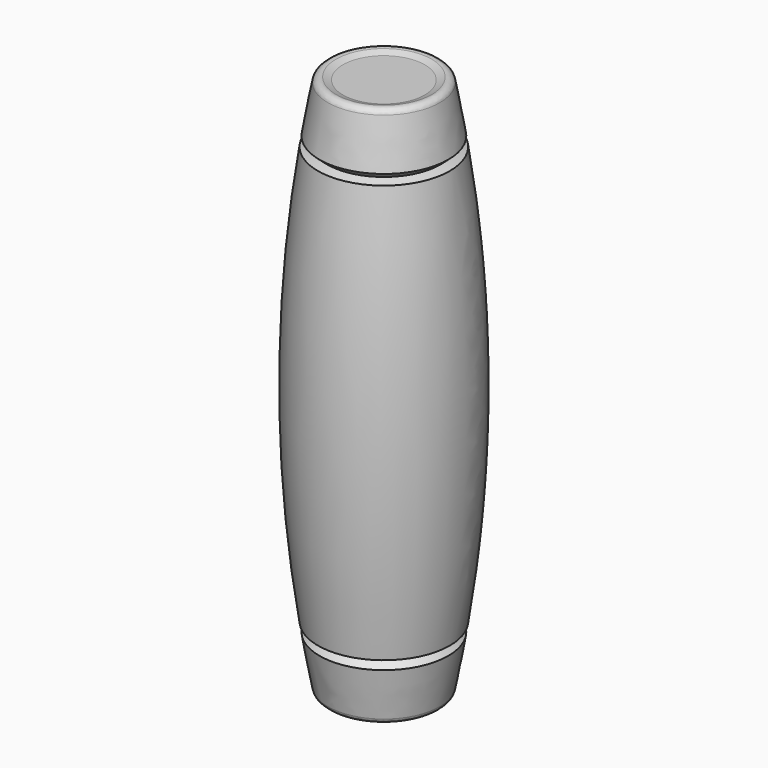
from build123d import *

# Parameters (mm, degrees)
F2_R = 1


with BuildPart() as f1:
    # F0 (on Front) → F1 (revolve)
    with BuildSketch(Plane.XZ):
        with BuildLine():
            Line((6.75, 0), (8.9949437628, -0.8157445242))
            ThreePointArc((8.9949437628, -0.8157445242), (13.5, 44.1842554758), (8.9949437628, 89.1842554758))
            Line((8.9949437628, 89.1842554758), (6.75, 88.3685109515))
            Line((6.75, 88.3685109515), (0, 88.3685109515))
            Line((0, 88.3685109515), (0, 0))
            Line((0, 0), (6.75, 0))
        make_face()
    revolve(axis=Axis((0, 0, 44.1842554758), (0, 0, 1)))

    # F2
    f2_edges = [f1.edges().sort_by_distance(p)[0] for p in [
        (-8.994944, 0, -0.815745),
        (-8.994944, 0, 89.184255),
    ]]
    fillet(f2_edges, radius=F2_R)

    # F3 (on Front) → F4 (revolve, cut)
    with BuildSketch(Plane.XZ):
        Polygon((17.6116488874, 76.3894766569), (14.7303857711, 83.846378142), (9.4051705673, 79.1429653764), align=None)
        Polygon((9.4051705673, 9.2255455751), (14.7303857711, 4.5221328095), (17.6116488874, 11.9790342946), align=None)
    revolve(axis=Axis((0, 0, 27.809754014), (0, 0, 1)), mode=Mode.SUBTRACT)


solid = f1.part
